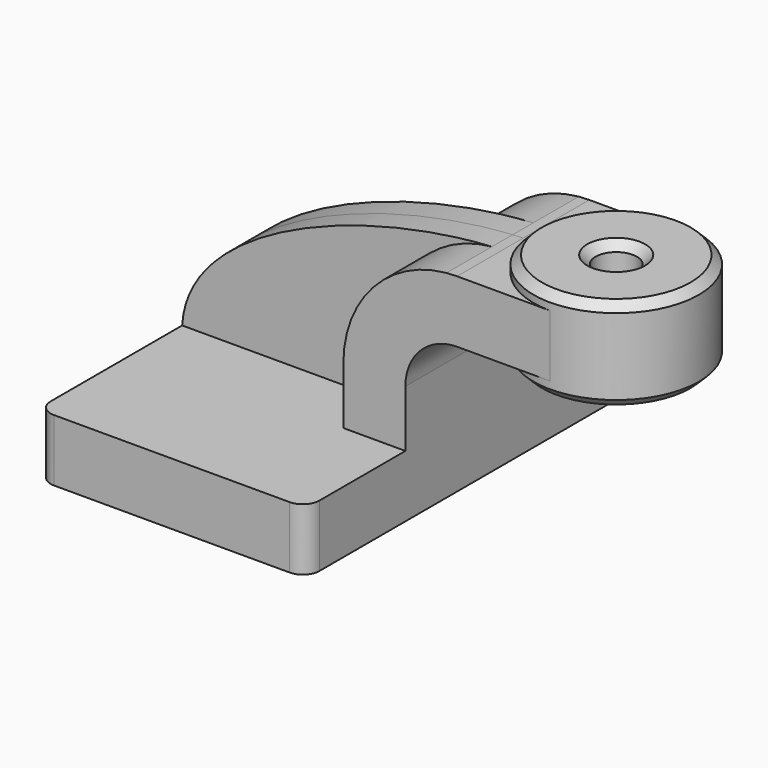
from build123d import *

# Parameters (mm, degrees)
F1_DEPTH = 63.5
F0_W     = 25.4
F0_H     = 19.05
F2_DEPTH = 25.4
F3_DEPTH = 7.9375
F5_R     = 5.08
F7_D     = 12.7
F8_SIZE  = 2.54


with BuildPart() as f1:
    # F0 (on Front) → F1 (new body, symmetric)
    with BuildSketch(Plane.XZ):
        Polygon((22.225, 9.525), (-41.275, 9.525), (-41.275, -9.525), (41.275, -9.525), (41.275, 9.525), align=None)
    extrude(amount=F1_DEPTH, both=True)

    # F0 (on Front) → F2 (join, symmetric)
    with BuildSketch(Plane.XZ):
        with BuildLine():
            Line((22.225, 27.0002), (22.225, 9.525))
            Line((22.225, 9.525), (41.275, 9.525))
            Line((41.275, 9.525), (41.275, 27.0002))
            ThreePointArc((41.275, 27.0002), (45.9246798487, 38.2255201513), (57.15, 42.8752))
            Line((57.15, 42.8752), (60.325, 42.8752))
            Line((60.325, 42.8752), (60.325, 61.9252))
            Line((60.325, 61.9252), (57.15, 61.9252))
            add(Edge.make_bspline(
                [(53.8854342407, 61.7722898912), (54.9842067368, 61.8365871986), (56.0728453275, 61.8876096574), (57.15, 61.9252)],
                knots=[108.5245810491, 108.5245810491, 108.5245810491, 108.5245810491, 111.5045361635, 111.5045361635, 111.5045361635, 111.5045361635], degree=3))
            ThreePointArc((53.8854342407, 61.7722898912), (31.3258777096, 50.5133948686), (22.225, 27.0002))
        make_face()
        with Locations((73.025, 52.4002)):
            Rectangle(F0_W, F0_H)
    extrude(amount=F2_DEPTH, both=True)

    # F0 (on Front) → F3 (join, symmetric)
    with BuildSketch(Plane.XZ):
        with BuildLine():
            add(Edge.make_bspline(
                [(-41.275, 9.525), (-39.5856284224, 39.4828766469), (13.870125209, 59.4306981306), (53.8854342407, 61.7722898912)],
                knots=[0, 0, 0, 0, 108.5245810491, 108.5245810491, 108.5245810491, 108.5245810491], degree=3))
            Line((-41.275, 9.525), (22.225, 9.525))
            Line((22.225, 9.525), (22.225, 27.0002))
            ThreePointArc((22.225, 27.0002), (31.3258777096, 50.5133948686), (53.8854342407, 61.7722898912))
        make_face()
    extrude(amount=F3_DEPTH, both=True)

    # F0 (on Front) → F4 (revolve)
    with BuildSketch(Plane.XZ):
        Polygon((85.725, 66.675), (85.725, 61.9252), (85.725, 42.8752), (85.725, 38.1), (111.125, 38.1), (111.125, 66.675), align=None)
    revolve(axis=Axis((85.725, 0, 52.3875), (0, 0, 1)))

    # F5
    f5_edges = [f1.edges().sort_by_distance(p)[0] for p in [
        (41.275, -63.5, 0),
        (-41.275, -63.5, 0),
        (41.275, 63.5, 0),
        (-41.275, 63.5, 0),
    ]]
    fillet(f5_edges, radius=F5_R)

    # F7 (through all)
    with Locations(Plane.XY.offset(66.675)):
        with Locations((85.725, 0)):
            Hole(F7_D / 2)

    # F8
    f8_edges = [f1.edges().sort_by_distance(p)[0] for p in [
        (60.325, 0, 66.675),
        (60.325, 0, 38.1),
        (79.375, 0, 66.675),
        (79.375, 0, 38.1),
    ]]
    chamfer(f8_edges, length=F8_SIZE)


solid = f1.part
